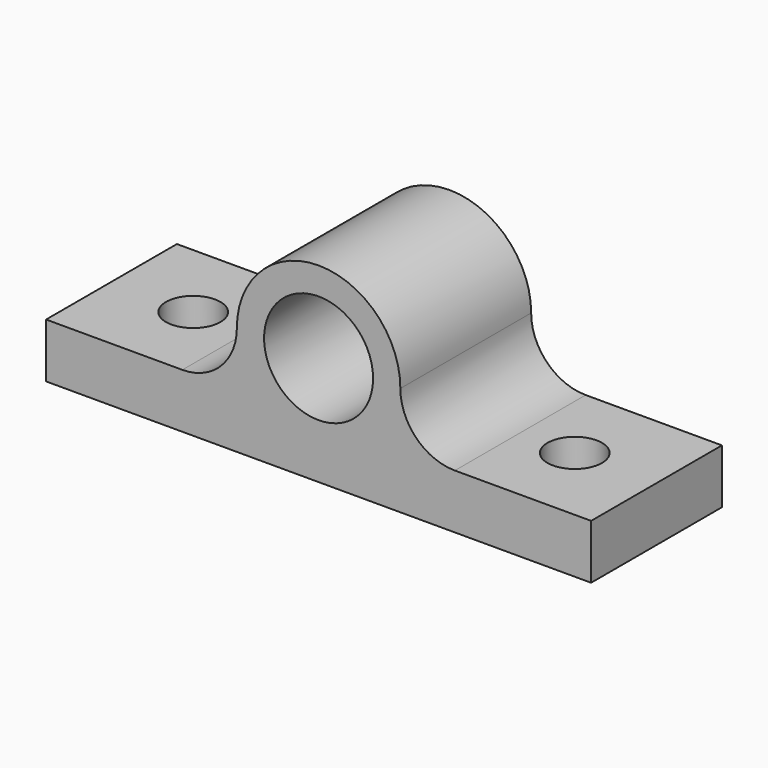
from build123d import *

# Parameters (mm, degrees)
F0_R     = 12.7
F1_DEPTH = 38.1
F2_R     = 6.35
F3_DEPTH = 25.4


# Not quite as in the source:
# - a feature names something its author has since deleted; it is built from what else it names


with BuildPart() as f1:
    # F0 (on Front) → F1 (new body)
    with BuildSketch(Plane.XZ):
        with BuildLine():
            Line((-39.8161155887, 12.7), (-39.8161155887, 0))
            Line((-39.8161155887, 0), (87.1838844113, 0))
            Line((87.1838844113, 0), (87.1838844113, 12.7))
            Line((87.1838844113, 12.7), (55.4338844113, 12.7))
            ThreePointArc((55.4338844113, 12.7), (46.4536282902, 16.4197438789), (42.7338844113, 25.4))
            ThreePointArc((42.7338844113, 25.4), (23.6838844113, 44.45), (4.6338844113, 25.4))
            ThreePointArc((4.6338844113, 25.4), (0.9141405324, 16.4197438789), (-8.0661155887, 12.7))
            Line((-8.0661155887, 12.7), (-39.8161155887, 12.7))
        make_face()
        with Locations((23.6838844113, 25.4)):
            Circle(F0_R, mode=Mode.SUBTRACT)
    extrude(amount=-F1_DEPTH)

    # F2 (on Top) → F3 (cut)
    with BuildSketch(Plane.XY):
        with Locations((-20.7661155887, 19.05)):
            Circle(F2_R)
        with Locations((68.1338844113, 19.05)):
            Circle(F2_R)
    extrude(amount=F3_DEPTH, mode=Mode.SUBTRACT)


solid = f1.part
